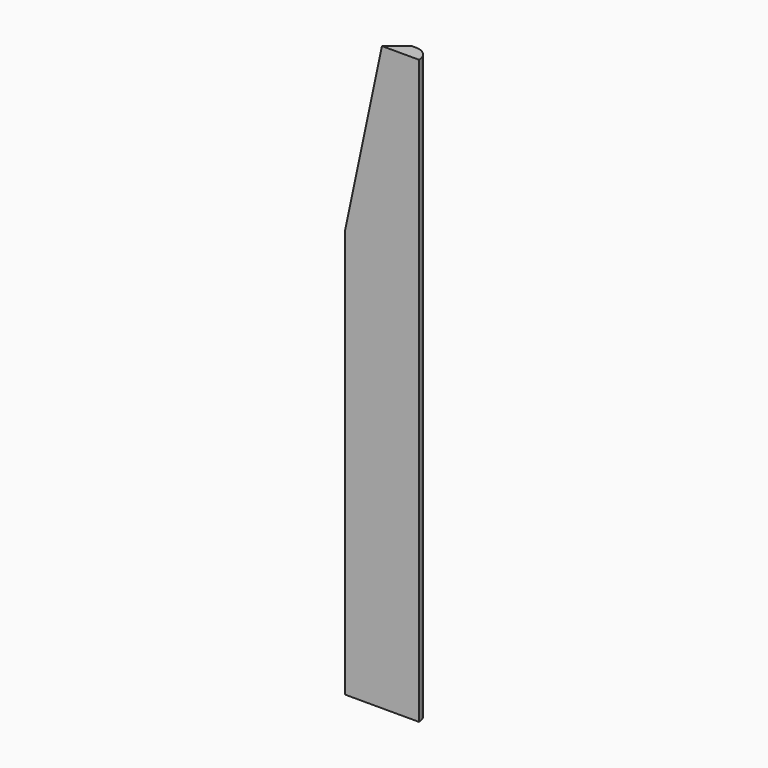
from build123d import *

# Parameters (mm, degrees)
F7_R = 2.49999


# Not quite as in the source:
# - a fillet or chamfer is up to 0.001 mm smaller than in the source, because OpenCascade refuses the exact size


with BuildPart() as f5:
    # F0 (on Top) → F5 section 0
    with BuildSketch(Plane.XY):
        Polygon((-6.35, -1.25), (6.35, -1.25), (6.35, 1.25), (0, 1.25), align=None)
    # F2 (on offset) → F5 section 1
    with BuildSketch(Plane.XY.offset(70)):
        Polygon((-6.35, -1.25), (6.35, -1.25), (6.35, 1.25), (0, 1.25), align=None)
    loft()

    # F2 (on offset) → F6 section 0
    with BuildSketch(Plane.XY.offset(70)):
        Polygon((-6.35, -1.25), (6.35, -1.25), (6.35, 1.25), (0, 1.25), align=None)
    # F4 (on offset) → F6 section 1
    with BuildSketch(Plane.XY.offset(100)):
        Polygon((0, -1.25), (6.35, -1.25), (6.35, 1.25), (3.175, 1.25), align=None)
    loft()

    # F7 (radius 2.5 in the source; OpenCascade refuses exactly that, so slightly less here)
    f7_edges = [f5.edges().sort_by_distance(p)[0] for p in [
        (6.35, 1.25, 50),
    ]]
    fillet(f7_edges, radius=F7_R)


solid = f5.part
